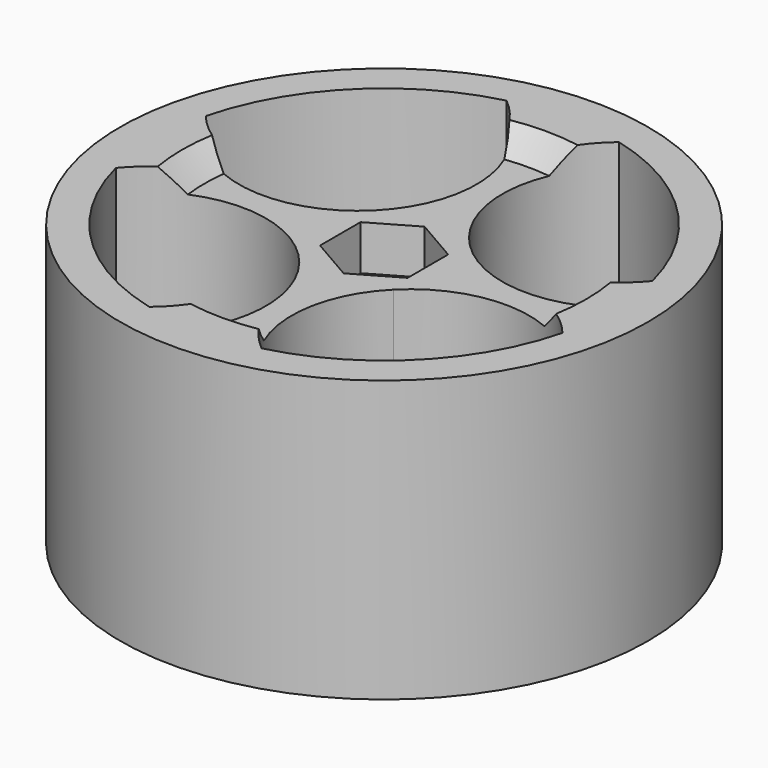
from build123d import *

# Parameters (mm, degrees)
F0_R      = 23.5
F0_R_2    = 22.5
F0_R_3    = 3
F1_DEPTH  = 25
F2_START  = 2
F0_R_4    = 2.75
F2_DEPTH  = 21
F2_FACE_R = 2.75
F4_DEPTH  = 6
F5_START  = 19
F5_DEPTH  = 6


# Not quite as in the source:
# - a fillet or chamfer that OpenCascade refuses, or shapes differently, is made with other operations: its cross-section is extruded or revolved along the edge and cut away or added


with BuildPart() as f1:
    # F0 (on Top) → F1 (new body)
    with BuildSketch(Plane.XY):
        Circle(F0_R)
        Circle(F0_R_2, mode=Mode.SUBTRACT)
        Circle(F0_R_2)
        with BuildLine():
            ThreePointArc((19.8808953521, 5), (20.3446351002, 2.5190916302), (20.5, 0))
            ThreePointArc((20.5, 0), (20.3446351002, -2.5190916302), (19.8808953521, -5))
            ThreePointArc((19.8808953521, -5), (14.4956890143, -14.4956890143), (5, -19.8808953521))
            ThreePointArc((5, -19.8808953521), (0, -20.5), (-5, -19.8808953521))
            ThreePointArc((-5, -19.8808953521), (-14.4956890143, -14.4956890143), (-19.8808953521, -5))
            ThreePointArc((-19.8808953521, -5), (-20.5, 0), (-19.8808953521, 5))
            ThreePointArc((-19.8808953521, 5), (-14.4956890143, 14.4956890143), (-5, 19.8808953521))
            ThreePointArc((-5, 19.8808953521), (0, 20.5), (5, 19.8808953521))
            ThreePointArc((5, 19.8808953521), (14.4956890143, 14.4956890143), (19.8808953521, 5))
        make_face(mode=Mode.SUBTRACT)
        with BuildLine():
            ThreePointArc((6, 0), (5.5432771953, 2.2961005937), (4.2426406878, 4.2426406864))
            ThreePointArc((4.2426406878, 4.2426406864), (7.8e-09, 6), (-4.2426406768, 4.2426406974))
            ThreePointArc((-4.2426406768, 4.2426406974), (-6, 7.9e-09), (-4.242640688, -4.2426406862))
            ThreePointArc((-4.242640688, -4.2426406862), (-1.21e-08, -6), (4.2426406709, -4.2426407033))
            ThreePointArc((4.2426406709, -4.2426407033), (5.5432771907, -2.2961006048), (6, 0))
        make_face()
        Polygon((-3.9, -2.2516660498), (-3.9, 2.2516660498), (0, 4.5033320997), (3.9, 2.2516660498), (3.9, -2.2516660498), (0, -4.5033320997), align=None, mode=Mode.SUBTRACT)
        with BuildLine():
            ThreePointArc((4.2426406878, 4.2426406864), (1.1585914251, 12.2294676794), (5, 19.8808953521))
            ThreePointArc((5, 19.8808953521), (0, 20.5), (-5, 19.8808953521))
            ThreePointArc((-5, 19.8808953521), (-1.1585914255, 12.2294676871), (-4.2426406768, 4.2426406974))
            ThreePointArc((-4.2426406768, 4.2426406974), (7.8e-09, 6), (4.2426406878, 4.2426406864))
        make_face()
        with BuildLine():
            ThreePointArc((19.8808953521, -5), (20.3446351002, -2.5190916302), (20.5, 0))
            ThreePointArc((20.5, 0), (20.3446351002, 2.5190916302), (19.8808953521, 5))
            ThreePointArc((19.8808953521, 5), (12.2294676803, 1.1585914252), (4.2426406878, 4.2426406864))
            ThreePointArc((4.2426406878, 4.2426406864), (5.5432771953, 2.2961005937), (6, 0))
            ThreePointArc((6, 0), (5.5432771907, -2.2961006048), (4.2426406709, -4.2426407033))
            ThreePointArc((4.2426406709, -4.2426407033), (12.2294676684, -1.1585914246), (19.8808953521, -5))
        make_face()
        with BuildLine():
            ThreePointArc((-5, -19.8808953521), (0, -20.5), (5, -19.8808953521))
            ThreePointArc((5, -19.8808953521), (1.1585914257, -12.2294676913), (4.2426406709, -4.2426407033))
            ThreePointArc((4.2426406709, -4.2426407033), (-1.21e-08, -6), (-4.242640688, -4.2426406862))
            ThreePointArc((-4.242640688, -4.2426406862), (-1.1585914251, -12.2294676792), (-5, -19.8808953521))
        make_face()
        with BuildLine():
            ThreePointArc((-4.242640688, -4.2426406862), (-6, 7.9e-09), (-4.2426406768, 4.2426406974))
            ThreePointArc((-4.2426406768, 4.2426406974), (-12.2294676726, 1.1585914248), (-19.8808953521, 5))
            ThreePointArc((-19.8808953521, 5), (-20.5, 0), (-19.8808953521, -5))
            ThreePointArc((-19.8808953521, -5), (-12.2294676805, -1.1585914252), (-4.242640688, -4.2426406862))
        make_face()
        Polygon((0, 4.5033320997), (-3.9, 2.2516660498), (-3.9, -2.2516660498), (0, -4.5033320997), (3.9, -2.2516660498), (3.9, 2.2516660498), align=None)
        Circle(F0_R_3, mode=Mode.SUBTRACT)
    extrude(amount=F1_DEPTH)

    # F0 (on Top) → F2 (join)
    with BuildSketch(Plane.XY.offset(F2_START)):
        Circle(F0_R_3)
        Circle(F0_R_4, mode=Mode.SUBTRACT)
    extrude(amount=F2_DEPTH)

    # F3: chamfer of 15 on 1 edges, made by hand


with BuildPart() as f3_tool2:
    # F3_s3 → F3_t4 (revolve)
    with BuildSketch(Plane.XZ):
        Polygon((18, 25), (3, 10), (3, 25), align=None)
    revolve(axis=Axis((0, 0, 25), (0, 0, 1)))

    split(bisect_by=Plane.XY.offset(23), keep=Keep.TOP)


with BuildPart() as f1_1:
    add(f1.part)

    # F3_t1: cut F3_tool2
    add(f3_tool2.part, mode=Mode.SUBTRACT)

    # F0 (on Top) + F2_face (on face) → F4 (cut)
    with BuildSketch(Plane.XY):
        Polygon((0, 4.5033320997), (-3.9, 2.2516660498), (-3.9, -2.2516660498), (0, -4.5033320997), (3.9, -2.2516660498), (3.9, 2.2516660498), align=None)
        Circle(F0_R_3, mode=Mode.SUBTRACT)
        Circle(F0_R_3)
        Circle(F0_R_4, mode=Mode.SUBTRACT)
    with BuildSketch(Plane.XY.offset(23)):
        with BuildLine():
            ThreePointArc((15.874798485, -1.9976919331), (16, 0), (15.874798485, 1.9976919331))
            ThreePointArc((15.874798485, 1.9976919331), (4.2426406871, 4.2426406871), (1.9976919331, 15.874798485))
            ThreePointArc((1.9976919331, 15.874798485), (0, 16), (-1.9976919331, 15.874798485))
            ThreePointArc((-1.9976919331, 15.874798485), (-4.2426406871, 4.2426406871), (-15.874798485, 1.9976919331))
            ThreePointArc((-15.874798485, 1.9976919331), (-16, 0), (-15.874798485, -1.9976919331))
            ThreePointArc((-15.874798485, -1.9976919331), (-4.2426406871, -4.2426406871), (-1.9976919331, -15.874798485))
            ThreePointArc((-1.9976919331, -15.874798485), (0, -16), (1.9976919331, -15.874798485))
            ThreePointArc((1.9976919331, -15.874798485), (4.2426406871, -4.2426406871), (15.874798485, -1.9976919331))
        make_face()
        Circle(F2_FACE_R, mode=Mode.SUBTRACT)
    extrude(amount=F4_DEPTH, mode=Mode.SUBTRACT)

    # F0 (on Top) → F5 (cut)
    with BuildSketch(Plane.XY.offset(F5_START)):
        Polygon((0, 4.5033320997), (-3.9, 2.2516660498), (-3.9, -2.2516660498), (0, -4.5033320997), (3.9, -2.2516660498), (3.9, 2.2516660498), align=None)
        Circle(F0_R_3, mode=Mode.SUBTRACT)
        Circle(F0_R_3)
        Circle(F0_R_4, mode=Mode.SUBTRACT)
    extrude(amount=F5_DEPTH, mode=Mode.SUBTRACT)


solid = f1_1.part
